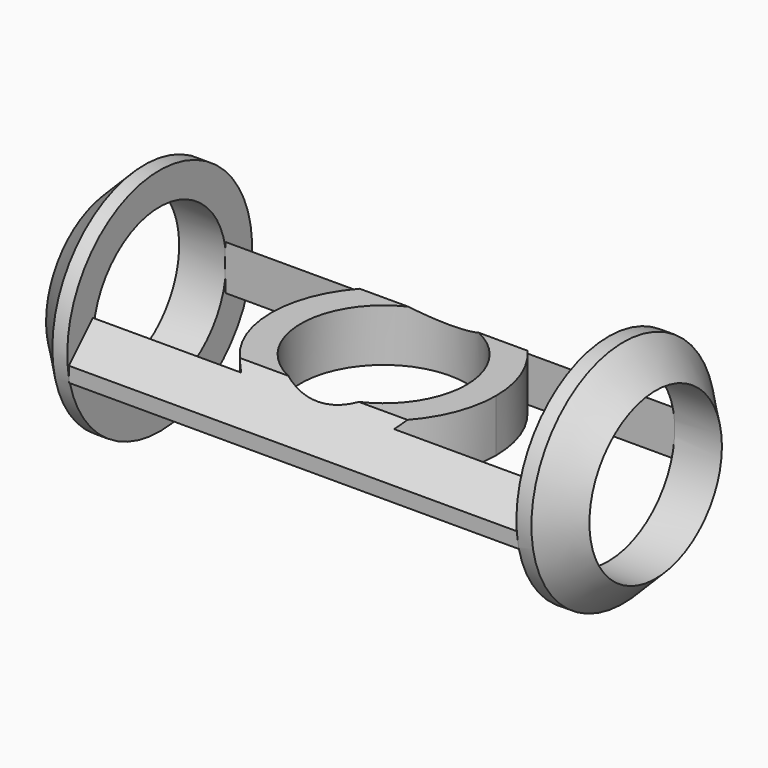
from build123d import *

# Parameters (mm, degrees)
F0_R        = 11.05
F1_DEPTH    = 7
F2_R        = 15.35
F2_R_2      = 11.05
F3_DEPTH    = 7
F4_R        = 15.35
F4_R_2      = 11.05
F5_DEPTH    = 7
F6_T4_DEPTH = 72.7584417561
F6_T9_DEPTH = 72.8584149398


# Not quite as in the source:
# - a fillet or chamfer that OpenCascade refuses, or shapes differently, is made with other operations: its cross-section is extruded or revolved along the edge and cut away or added


with BuildPart() as f1:
    # F0 (on Top) → F1 (new body)
    with BuildSketch(Plane.XY):
        with BuildLine():
            ThreePointArc((10.1980390272, -11), (13.7471921753, -6.0012254829), (15, 0))
            ThreePointArc((15, 0), (13.7471921753, 6.0012254829), (10.1980390272, 11))
            ThreePointArc((10.1980390272, 11), (5.4772255751, 13.9642400438), (0, 15))
            ThreePointArc((0, 15), (-5.4772255751, 13.9642400438), (-10.1980390272, 11))
            ThreePointArc((-10.1980390272, 11), (-15, 0), (-10.1980390272, -11))
            ThreePointArc((-10.1980390272, -11), (-5.4772255751, -13.9642400438), (0, -15))
            ThreePointArc((0, -15), (5.4772255751, -13.9642400438), (10.1980390272, -11))
        make_face()
        Circle(F0_R, mode=Mode.SUBTRACT)
        with BuildLine():
            ThreePointArc((0, 15), (5.4772255751, 13.9642400438), (10.1980390272, 11))
            Line((10.1980390272, 11), (30, 11))
            Line((30, 11), (30, 15))
            Line((30, 15), (0, 15))
        make_face()
        with BuildLine():
            Line((30, -11), (10.1980390272, -11))
            ThreePointArc((10.1980390272, -11), (5.4772255751, -13.9642400438), (0, -15))
            Line((0, -15), (30, -15))
            Line((30, -15), (30, -11))
        make_face()
        with BuildLine():
            ThreePointArc((-10.1980390272, 11), (-5.4772255751, 13.9642400438), (0, 15))
            Line((0, 15), (-30, 15))
            Line((-30, 15), (-29.9866729691, 11))
            Line((-29.9866729691, 11), (-10.1980390272, 11))
        make_face()
        with BuildLine():
            Line((-30, -15), (0, -15))
            ThreePointArc((0, -15), (-5.4772255751, -13.9642400438), (-10.1980390272, -11))
            Line((-10.1980390272, -11), (-29.9866702422, -11))
            Line((-29.9866702422, -11), (-30, -15))
        make_face()
    extrude(amount=F1_DEPTH)

    # F2 (on face) → F3 (join)
    with BuildSketch(Plane(origin=(-29.9496808123, 0.0998054981, 0), x_dir=(-0.003332421, -0.9999944475, 0), z_dir=(-0.9999944475, 0.003332421, 0))):
        with Locations((0, 3.5)):
            Circle(F2_R)
        with Locations((0, 3.5)):
            Circle(F2_R_2, mode=Mode.SUBTRACT)
    extrude(amount=F3_DEPTH)

    # F4 (on face) → F5 (join)
    with BuildSketch(Plane.YZ.offset(30)):
        with Locations((0, 3.5)):
            Circle(F4_R)
        with Locations((0, 3.5)):
            Circle(F4_R_2, mode=Mode.SUBTRACT)
    extrude(amount=F5_DEPTH)

    # F6: chamfer of 5 on 4 edges, made by hand


with BuildPart() as f6_tool2:
    # F6_s3 → F6_t4 (new body)
    with BuildSketch(Plane.YZ.offset(30)):
        Polygon((10, 7), (15, 2), (15, 7), align=None)
    extrude(amount=-F6_T4_DEPTH)

    split(bisect_by=Plane(origin=(-29.9496808123, 0.0998054981, 0), x_dir=(0, 0, 1), z_dir=(0.9999944475, -0.003332421, 0)), keep=Keep.TOP)


with BuildPart() as f1_1:
    add(f1.part)

    # F6_t1: cut F6_tool2
    add(f6_tool2.part, mode=Mode.SUBTRACT)


with BuildPart() as f6_tool7:
    # F6_s8 → F6_t9 (new body)
    with BuildSketch(Plane.YZ.offset(-42.8584149398)):
        Polygon((-10, 7), (-15, 2), (-15, 7), align=None)
    extrude(amount=F6_T9_DEPTH)

    split(bisect_by=Plane(origin=(-29.9496808123, 0.0998054981, 0), x_dir=(0, 0, 1), z_dir=(0.9999944475, -0.003332421, 0)), keep=Keep.TOP)


with BuildPart() as f1_2:
    add(f1_1.part)

    # F6_t6: cut F6_tool7
    add(f6_tool7.part, mode=Mode.SUBTRACT)

    # F6_s11 → F6_t12 (revolve, cut)
    with BuildSketch(Plane.XY.offset(3.5)):
        Polygon((32, 15.35), (37, 10.35), (37, 15.35), align=None)
    revolve(axis=Axis((37, 0, 3.5), (1, 0, 0)), mode=Mode.SUBTRACT)

    # F6_s13 → F6_t14 (revolve, cut)
    with BuildSketch(Plane.XY.offset(3.5)):
        Polygon((-32.0008223689, -15.2434444286), (-36.9841325015, -10.2268100865), (-37.0007946063, -15.2267823238), align=None)
    revolve(axis=Axis((-36.9496419446, 0.1231324448, 3.5), (-0.9999944475, 0.003332421, 0)), mode=Mode.SUBTRACT)


solid = f1_2.part
